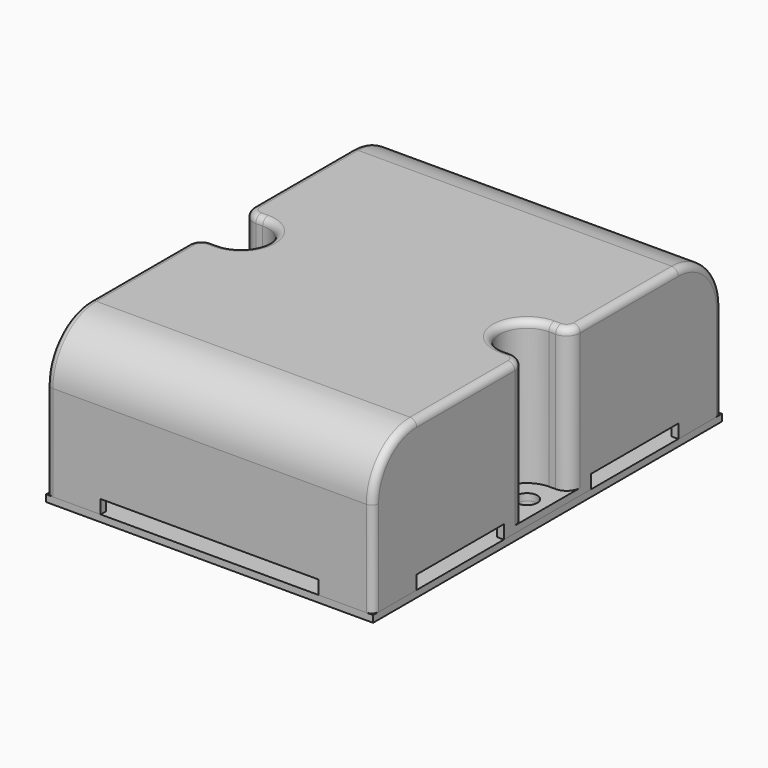
from build123d import *

# Parameters (mm, degrees)
F0_W      = 76.2
F0_H      = 101.6
F1_DEPTH  = 1.5875
F2_R      = 2.38125
F3_DEPTH  = 1.5885
F4_W      = 76.2
F4_H      = 101.6
F5_DEPTH  = 34.925
F6_R      = 12.7
F8_DEPTH  = 36.5135
F9_R      = 3.175
F10_T     = -1.5875
F11_R     = 1.5875
F12_R     = 0.79375
F14_DEPTH = 1.5875
F15_R     = 2.38125
F16_DEPTH = 25.4
F18_DEPTH = 3.175


with BuildPart() as f1:
    # F0 (on Top) → F1 (new body)
    with BuildSketch(Plane.XY):
        Rectangle(F0_W, F0_H)
    extrude(amount=-F1_DEPTH)

    # F2 (on face) → F3 (cut, through all)
    with BuildSketch(Plane.XY):
        with Locations((33.3375, 0)):
            Circle(F2_R)
        with Locations((-33.3375, 0)):
            Circle(F2_R)
    extrude(amount=-F3_DEPTH, mode=Mode.SUBTRACT)


with BuildPart() as f5:
    # F4 (on face) → F5 (new body)
    with BuildSketch(Plane.XY):
        Rectangle(F4_W, F4_H)
    extrude(amount=F5_DEPTH)

    # F6
    f6_edges = [f5.edges().sort_by_distance(p)[0] for p in [
        (0, -50.8, 34.925),
        (0, 50.8, 34.925),
    ]]
    fillet(f6_edges, radius=F6_R)

    # F7 (on face) → F8 (cut, through all)
    with BuildSketch(Plane.XY.offset(34.925)):
        with BuildLine():
            Line((-33.3375, 6.35), (-38.1, 6.35))
            Line((-38.1, 6.35), (-38.1, -6.35))
            Line((-38.1, -6.35), (-33.3375, -6.35))
            ThreePointArc((-33.3375, -6.35), (-26.9875, 0), (-33.3375, 6.35))
        make_face()
        with BuildLine():
            Line((38.1, -6.35), (38.1, 6.35))
            Line((38.1, 6.35), (33.3375, 6.35))
            ThreePointArc((33.3375, 6.35), (26.9875, 0), (33.3375, -6.35))
            Line((33.3375, -6.35), (38.1, -6.35))
        make_face()
    extrude(amount=-F8_DEPTH, mode=Mode.SUBTRACT)

    # F9
    f9_edges = [f5.edges().sort_by_distance(p)[0] for p in [
        (38.1, -6.35, 17.4625),
        (38.1, 6.35, 17.4625),
        (-38.1, -6.35, 17.4625),
        (-38.1, 6.35, 17.4625),
    ]]
    fillet(f9_edges, radius=F9_R)

    # F10
    f10_openings = [f5.faces().sort_by_distance(p)[0] for p in [
        (0, 0, 0),
    ]]
    offset(amount=F10_T, openings=f10_openings)

    # F11
    f11_edges = [f5.edges().sort_by_distance(p)[0] for p in [
        (-38.1, 50.8, 11.1125),
        (38.1, 50.8, 11.1125),
        (38.1, -50.8, 11.1125),
        (38.1, -23.8125, 34.925),
        (38.1, -47.080256, 31.205256),
        (37.170064, -7.279936, 34.925),
        (-38.1, -50.8, 11.1125),
        (-38.1, -23.8125, 34.925),
        (-37.170064, -7.279936, 34.925),
        (-34.13125, -6.35, 34.925),
        (-26.9875, 0, 34.925),
        (-34.13125, 6.35, 34.925),
        (34.13125, -6.35, 34.925),
        (-37.170064, 7.279936, 34.925),
        (26.9875, 0, 34.925),
        (-38.1, 23.8125, 34.925),
        (34.13125, 6.35, 34.925),
        (37.170064, 7.279936, 34.925),
        (38.1, 23.8125, 34.925),
        (-38.1, -47.080256, 31.205256),
        (-38.1, 47.080256, 31.205256),
        (38.1, 47.080256, 31.205256),
    ]]
    fillet(f11_edges, radius=F11_R)

    # F12
    f12_edges = [f5.edges().sort_by_distance(p)[0] for p in [
        (-36.5125, 49.2125, 11.1125),
        (36.5125, 49.2125, 11.1125),
        (-36.5125, -23.8125, 33.3375),
        (-36.5125, -45.957724, 30.082724),
        (-36.5125, -49.2125, 11.1125),
        (-36.047532, -8.402468, 33.3375),
        (-34.13125, -7.9375, 33.3375),
        (-25.4, 0, 33.3375),
        (-34.13125, 7.9375, 33.3375),
        (-36.047532, 8.402468, 33.3375),
        (-36.5125, 45.957724, 30.082724),
        (-36.5125, 23.8125, 33.3375),
        (36.5125, 23.8125, 33.3375),
        (36.5125, 45.957724, 30.082724),
        (36.047532, 8.402468, 33.3375),
        (34.13125, 7.9375, 33.3375),
        (25.4, 0, 33.3375),
        (34.13125, -7.9375, 33.3375),
        (36.047532, -8.402468, 33.3375),
        (36.5125, -49.2125, 11.1125),
        (36.5125, -45.957724, 30.082724),
        (36.5125, -23.8125, 33.3375),
    ]]
    fillet(f12_edges, radius=F12_R)

    # F13 (on face) → F14 (join)
    with BuildSketch(Plane(origin=(0, 0, 0), x_dir=(1, 0, 0), z_dir=(0, 0, -1))):
        with BuildLine():
            ThreePointArc((-34.925, 6.35), (-37.1700640303, 7.2799359697), (-38.1, 9.525))
            Line((-38.1, 9.525), (-38.1, -9.525))
            ThreePointArc((-38.1, -9.525), (-37.1700640303, -7.2799359697), (-34.925, -6.35))
            Line((-34.925, -6.35), (-33.3375, -6.35))
            ThreePointArc((-33.3375, -6.35), (-26.9875, 0), (-33.3375, 6.35))
            Line((-33.3375, 6.35), (-34.925, 6.35))
        make_face()
        with BuildLine():
            ThreePointArc((38.1, 9.525), (37.1700640303, 7.2799359697), (34.925, 6.35))
            Line((34.925, 6.35), (33.3375, 6.35))
            ThreePointArc((33.3375, 6.35), (26.9875, 0), (33.3375, -6.35))
            Line((33.3375, -6.35), (34.925, -6.35))
            ThreePointArc((34.925, -6.35), (37.1700640303, -7.2799359697), (38.1, -9.525))
            Line((38.1, -9.525), (38.1, 9.525))
        make_face()
    extrude(amount=-F14_DEPTH)

    # F15 (on face) → F16 (cut)
    with BuildSketch(Plane(origin=(0, 0, 0), x_dir=(1, 0, 0), z_dir=(0, 0, -1))):
        with Locations((-33.3375, 0)):
            Circle(F15_R)
        with Locations((33.3375, 0)):
            Circle(F15_R)
    extrude(amount=-F16_DEPTH, mode=Mode.SUBTRACT)

    # F17 (on face) → F18 (cut)
    with BuildSketch(Plane(origin=(0, 0, 0), x_dir=(1, 0, 0), z_dir=(0, 0, -1))):
        Polygon((25.4, 63.5), (-25.4, 63.5), (-25.4, 38.1), (-50.8, 38.1), (-50.8, 12.7), (50.8, 12.7), (50.8, 38.1), (25.4, 38.1), align=None)
        Polygon((25.4, -63.5), (25.4, -38.1), (50.8, -38.1), (50.8, -12.7), (-50.8, -12.7), (-50.8, -38.1), (-25.4, -38.1), (-25.4, -63.5), align=None)
    extrude(amount=-F18_DEPTH, mode=Mode.SUBTRACT)


solid = Compound([f1.part, f5.part])
